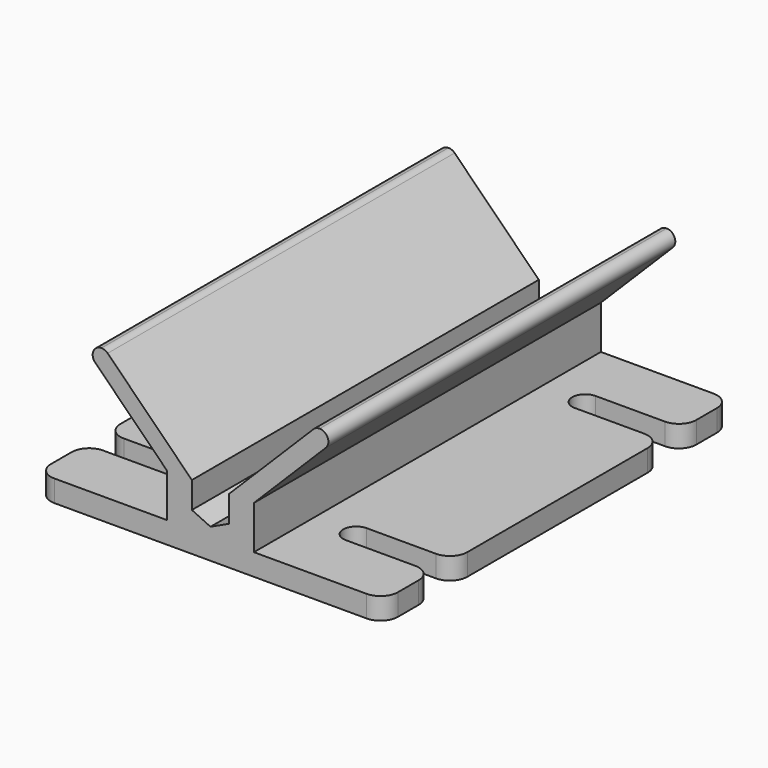
from build123d import *

# Parameters (mm, degrees)
F0_W     = 101.6
F0_H     = 44.45
F1_DEPTH = 63.5
F3_DEPTH = 127.001
F5_DEPTH = 127.001
F6_R     = 2.54
F8_DEPTH = 6.35
F9_R     = 5.08


# Not quite as in the source:
# - a pattern or mirror of a feature is missing from the dataset's text; its kind, count and spacing are read off the source's solid


with BuildPart() as f1:
    # F0 (on Front) → F1 (new body, symmetric)
    with BuildSketch(Plane.XZ):
        Rectangle(F0_W, F0_H)
    extrude(amount=F1_DEPTH, both=True)

    # F2 (on face) → F3 (cut, through all)
    with BuildSketch(Plane.XZ.offset(63.5)):
        Polygon((-50.8, -15.875), (-12.7, -15.875), (-12.7, -3.175), (-38.1, 22.225), (-50.8, 22.225), align=None)
    f3 = extrude(amount=-F3_DEPTH, mode=Mode.SUBTRACT)

    # F3_copies: F3 across plane
    add(f3.mirror(Plane(origin=(0, 0, 0), x_dir=(0, 0, 1), z_dir=(1, 0, 0))), mode=Mode.SUBTRACT)

    # F4 (on face) → F5 (cut, through all)
    with BuildSketch(Plane.XZ.offset(63.5)):
        Polygon((30.861, 22.225), (-30.861, 22.225), (-5.461, -3.175), (-5.461, -10.8996083293), (0, -13.4461144505), (5.461, -10.8996083293), (5.461, -3.175), align=None)
    extrude(amount=-F5_DEPTH, mode=Mode.SUBTRACT)

    # F6
    f6_edges = [f1.edges().sort_by_distance(p)[0] for p in [
        (-38.1, 0, 22.225),
        (-30.861, 0, 22.225),
        (30.861, 0, 22.225),
        (38.1, 0, 22.225),
    ]]
    fillet(f6_edges, radius=F6_R)

    # F7 (on face) → F8 (cut, through all)
    with BuildSketch(Plane(origin=(0, 0, -22.225), x_dir=(1, 0, 0), z_dir=(0, 0, -1))):
        with BuildLine():
            Line((-25.4, 45.72), (-50.8, 45.72))
            Line((-50.8, 45.72), (-50.8, 38.1))
            Line((-50.8, 38.1), (-25.4, 38.1))
            ThreePointArc((-25.4, 38.1), (-21.59, 41.91), (-25.4, 45.72))
        make_face()
        with BuildLine():
            Line((-25.4, -38.1), (-50.8, -38.1))
            Line((-50.8, -38.1), (-50.8, -45.72))
            Line((-50.8, -45.72), (-25.4, -45.72))
            ThreePointArc((-25.4, -45.72), (-21.59, -41.91), (-25.4, -38.1))
        make_face()
    f8 = extrude(amount=-F8_DEPTH, mode=Mode.SUBTRACT)

    # F8_copies: F8 across plane
    add(f8.mirror(Plane(origin=(0, 0, 0), x_dir=(0, 0, 1), z_dir=(1, 0, 0))), mode=Mode.SUBTRACT)

    # F9
    f9_edges = [f1.edges().sort_by_distance(p)[0] for p in [
        (-50.8, -63.5, -19.05),
        (-50.8, 63.5, -19.05),
        (50.8, -63.5, -19.05),
        (50.8, 63.5, -19.05),
        (-50.8, -45.72, -19.05),
        (-50.8, 38.1, -19.05),
        (-50.8, 45.72, -19.05),
        (-50.8, -38.1, -19.05),
        (50.8, 45.72, -19.05),
        (50.8, -45.72, -19.05),
        (50.8, -38.1, -19.05),
        (50.8, 38.1, -19.05),
    ]]
    fillet(f9_edges, radius=F9_R)


solid = f1.part
